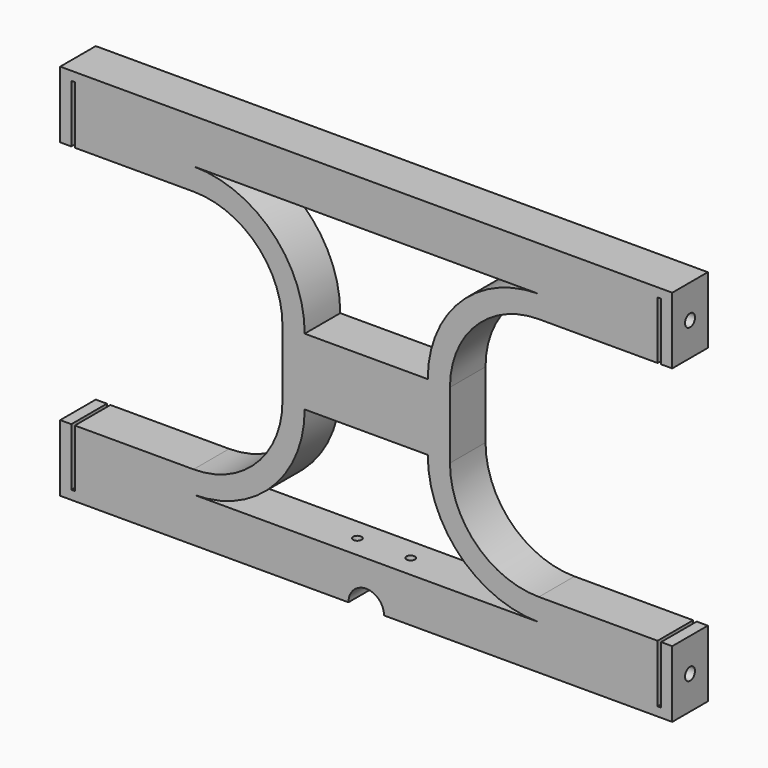
from build123d import *

# Parameters (mm, degrees)
F1_DEPTH  = 12.7
F2_W      = 1.016
F2_H      = 102.87
F3_DEPTH  = 25.4
F4_R      = 5.08
F5_DEPTH  = 25.4
F6_R      = 1.21539
F7_DEPTH  = 25.4
F8_R      = 1.397
F9_DEPTH  = 25.4
F10_R     = 1.397
F11_DEPTH = 19.05
F12_R     = 1.778
F13_DEPTH = 3.175
F15_DEPTH = 25.4
F16_W     = 12.7
F16_H     = 19.05
F17_DEPTH = 38.1


# Not quite as in the source:
# - a pattern or mirror of a feature is missing from the dataset's text; its kind, count and spacing are read off the source's solid


with BuildPart() as f1:
    # F0 (on Front) → F1 (new body)
    with BuildSketch(Plane.XZ):
        with BuildLine():
            Line((87.4268, 34.925), (87.4268, 53.975))
            Line((87.4268, 53.975), (0, 53.975))
            Line((0, 53.975), (-87.4268, 53.975))
            Line((-87.4268, 53.975), (-87.4268, 34.925))
            Line((-87.4268, 34.925), (-49.3268, 34.925))
            ThreePointArc((-49.3268, 34.925), (-31.3662877579, 27.4855122421), (-23.9268, 9.525))
            Line((-23.9268, 9.525), (-23.9268, -9.525))
            ThreePointArc((-23.9268, -9.525), (-31.3662877579, -27.4855122421), (-49.3268, -34.925))
            Line((-49.3268, -34.925), (-87.4268, -34.925))
            Line((-87.4268, -34.925), (-87.4268, -53.975))
            Line((-87.4268, -53.975), (87.4268, -53.975))
            Line((87.4268, -53.975), (87.4268, -34.925))
            Line((87.4268, -34.925), (49.3268, -34.925))
            ThreePointArc((49.3268, -34.925), (31.3662877579, -27.4855122421), (23.9268, -9.525))
            Line((23.9268, -9.525), (23.9268, 9.525))
            ThreePointArc((23.9268, 9.525), (31.3662877579, 27.4855122421), (49.3268, 34.925))
            Line((49.3268, 34.925), (87.4268, 34.925))
        make_face()
    extrude(amount=F1_DEPTH)

    # F2 (on face) → F3 (cut)
    with BuildSketch(Plane.XZ.offset(12.7)):
        with Locations((-83.7438, 0)):
            Rectangle(F2_W, F2_H)
        with Locations((83.7438, 0)):
            Rectangle(F2_W, F2_H)
    extrude(amount=-F3_DEPTH, mode=Mode.SUBTRACT)

    # F4 (on face) → F5 (cut)
    with BuildSketch(Plane.XZ.offset(12.7)):
        with Locations((0, -53.975)):
            Circle(F4_R)
    extrude(amount=-F5_DEPTH, mode=Mode.SUBTRACT)

    # F6 (on face) → F7 (cut)
    with BuildSketch(Plane(origin=(0, 0, -53.975), x_dir=(1, 0, 0), z_dir=(0, 0, -1))):
        with Locations((-7.62, 6.35)):
            Circle(F6_R)
        with Locations((7.62, 6.35)):
            Circle(F6_R)
    extrude(amount=-F7_DEPTH, mode=Mode.SUBTRACT)

    # F8 (on face) → F9 (cut)
    with BuildSketch(Plane.YZ.offset(87.4268)):
        with Locations((-6.35, 44.45)):
            Circle(F8_R)
        with Locations((-6.35, -44.45)):
            Circle(F8_R)
    extrude(amount=-F9_DEPTH, mode=Mode.SUBTRACT)

    # F10 (on face) → F11 (cut)
    with BuildSketch(Plane(origin=(-87.4268, 0, 0), x_dir=(0, -1, 0), z_dir=(-1, 0, 0))):
        with Locations((6.35, 44.45)):
            Circle(F10_R)
        with Locations((6.35, -44.45)):
            Circle(F10_R)
    extrude(amount=-F11_DEPTH, mode=Mode.SUBTRACT)

    # F12 (on face) → F13 (cut)
    with BuildSketch(Plane.YZ.offset(87.4268)):
        with Locations((-6.35, 44.45)):
            Circle(F12_R)
        with Locations((-6.35, -44.45)):
            Circle(F12_R)
    f13 = extrude(amount=-F13_DEPTH, mode=Mode.SUBTRACT)

    # F13_copies: F13 across plane
    add(f13.mirror(Plane(origin=(0, 0, 0), x_dir=(0, 0, -1), z_dir=(-1, 0, 0))), mode=Mode.SUBTRACT)

    # F14 (on face) → F15 (cut)
    with BuildSketch(Plane.XZ.offset(12.7)):
        with BuildLine():
            ThreePointArc((-17.5768, -9.525), (-26.8761596973, -31.9756403027), (-49.3268, -41.275))
            Line((-49.3268, -41.275), (49.3268, -41.275))
            ThreePointArc((49.3268, -41.275), (26.8761596973, -31.9756403027), (17.5768, -9.525))
            Line((17.5768, -9.525), (17.5768, 9.525))
            ThreePointArc((17.5768, 9.525), (26.8761596973, 31.9756403027), (49.3268, 41.275))
            Line((49.3268, 41.275), (-49.3268, 41.275))
            ThreePointArc((-49.3268, 41.275), (-26.8761596973, 31.9756403027), (-17.5768, 9.525))
            Line((-17.5768, 9.525), (-17.5768, -9.525))
        make_face()
    extrude(amount=-F15_DEPTH, mode=Mode.SUBTRACT)

    # F16 (on face) → F17 (join)
    with BuildSketch(Plane.YZ.offset(-17.5768)):
        with Locations((-6.35, 0)):
            Rectangle(F16_W, F16_H)
    extrude(amount=F17_DEPTH)


solid = f1.part
